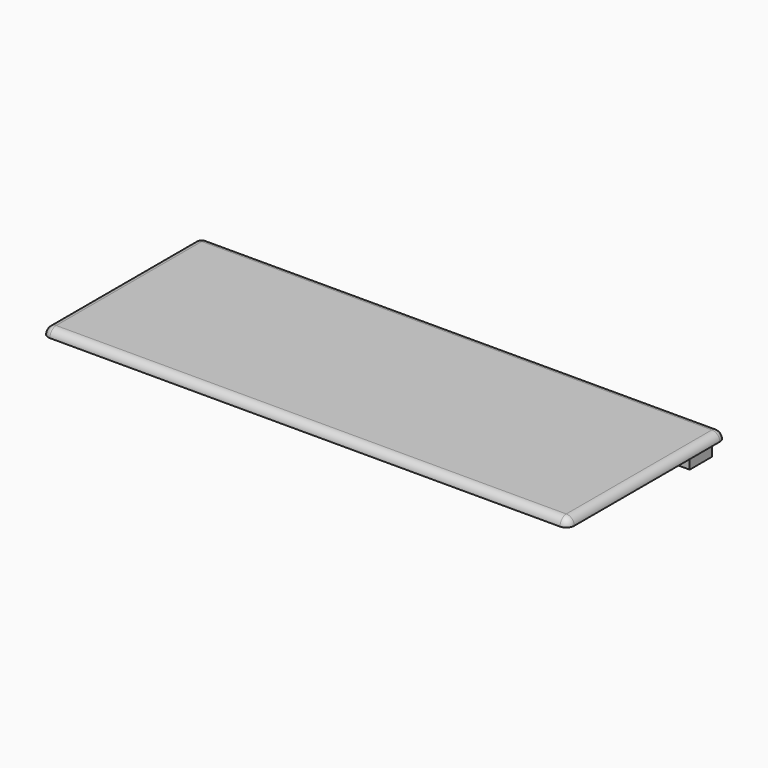
from build123d import *

# Parameters (mm, degrees)
F0_W     = 133
F0_H     = 50
F1_DEPTH = 2
F2_W     = 15
F2_H     = 7
F3_DEPTH = 4
F4_R     = 1.99999


# Not quite as in the source:
# - a fillet or chamfer is up to 0.001 mm smaller than in the source, because OpenCascade refuses the exact size


with BuildPart() as f1:
    # F0 (on Top) → F1 (new body)
    with BuildSketch(Plane.XY):
        Rectangle(F0_W, F0_H)
    extrude(amount=F1_DEPTH)

    # F2 (on face) → F3 (join)
    with BuildSketch(Plane(origin=(0, 0, 0), x_dir=(1, 0, 0), z_dir=(0, 0, -1))):
        with Locations((57, -19.5)):
            Rectangle(F2_W, F2_H)
    extrude(amount=F3_DEPTH)

    # F4 (radius 2 in the source; OpenCascade refuses exactly that, so slightly less here)
    f4_edges = [f1.edges().sort_by_distance(p)[0] for p in [
        (66.5, 25, 1),
        (66.5, -25, 1),
        (-66.5, 25, 1),
        (-66.5, -25, 1),
        (66.5, 0, 2),
        (0, 25, 2),
        (-66.5, 0, 2),
        (0, -25, 2),
    ]]
    fillet(f4_edges, radius=F4_R)


solid = f1.part
